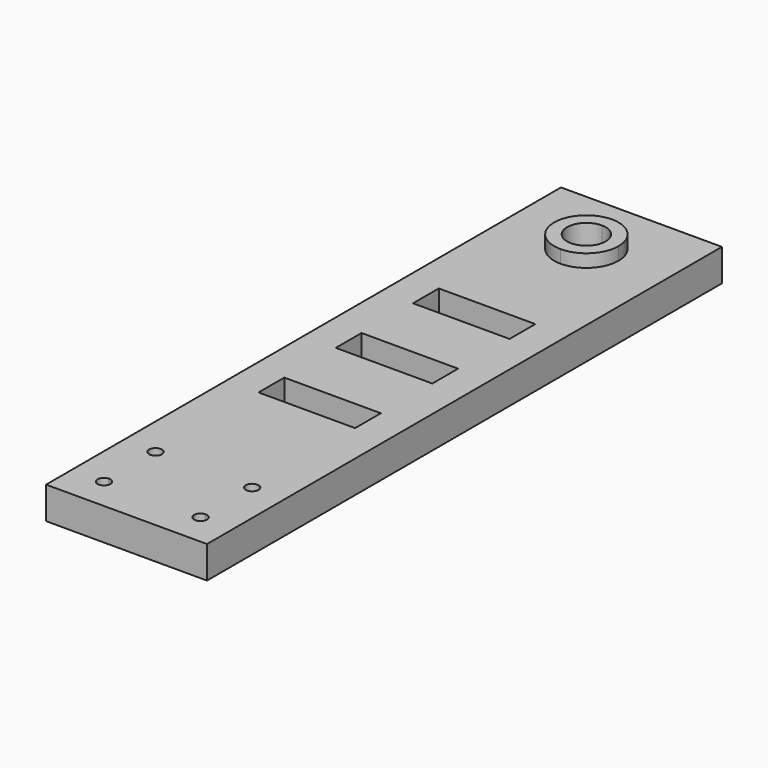
from build123d import *

# Parameters (mm, degrees)
F1_DEPTH = 5
F2_DEPTH = 7
F3_DEPTH = 1


with BuildPart() as f1:
    # F0 (on Top) → F1 (new body)
    with BuildSketch(Plane.XY):
        with BuildLine():
            Line((-12.5, -50), (0, -50))
            Line((0, -50), (0, -45))
            Line((0, -45), (-6.5, -45))
            ThreePointArc((-6.5, -45), (-8.2071067812, -45.7071067812), (-7.5, -44))
            Line((-7.5, -44), (-7.5, -35.9886))
            ThreePointArc((-7.5, -35.9886), (-8.2071067812, -34.2814932188), (-6.5, -34.9886))
            Line((-6.5, -34.9886), (0, -34.9886))
            Line((0, -34.9886), (0, -14.9886))
            Line((0, -14.9886), (-7.5, -14.9886))
            Line((-7.5, -14.9886), (-7.5, -9.9886))
            Line((-7.5, -9.9886), (0, -9.9886))
            Line((0, -9.9886), (0, 0.0114))
            Line((0, 0.0114), (-7.5, 0.0114))
            Line((-7.5, 0.0114), (-7.5, 5.0114))
            Line((-7.5, 5.0114), (0, 5.0114))
            Line((0, 5.0114), (0, 15.0114))
            Line((0, 15.0114), (-7.5, 15.0114))
            Line((-7.5, 15.0114), (-7.5, 20.0114))
            Line((-7.5, 20.0114), (0, 20.0114))
            Line((0, 20.0114), (0, 34.3023235092))
            ThreePointArc((0, 34.3023235092), (-5, 39.3023235092), (0, 44.3023235092))
            Line((0, 44.3023235092), (0, 50))
            Line((0, 50), (-12.5, 50))
            Line((-12.5, 50), (-12.5, -50))
        make_face()
        with BuildLine():
            Line((0, -50), (12.5, -50))
            Line((12.5, -50), (12.5, 50))
            Line((12.5, 50), (0, 50))
            Line((0, 50), (0, 44.3023235092))
            ThreePointArc((0, 44.3023235092), (3.5355339059, 42.8378574152), (5, 39.3023235092))
            ThreePointArc((5, 39.3023235092), (3.5355339059, 35.7667896033), (0, 34.3023235092))
            Line((0, 34.3023235092), (0, 20.0114))
            Line((0, 20.0114), (7.5, 20.0114))
            Line((7.5, 20.0114), (7.5, 15.0114))
            Line((7.5, 15.0114), (0, 15.0114))
            Line((0, 15.0114), (0, 5.0114))
            Line((0, 5.0114), (7.5, 5.0114))
            Line((7.5, 5.0114), (7.5, 0.0114))
            Line((7.5, 0.0114), (0, 0.0114))
            Line((0, 0.0114), (0, -9.9886))
            Line((0, -9.9886), (7.5, -9.9886))
            Line((7.5, -9.9886), (7.5, -14.9886))
            Line((7.5, -14.9886), (0, -14.9886))
            Line((0, -14.9886), (0, -34.9886))
            Line((0, -34.9886), (6.5, -34.9886))
            ThreePointArc((6.5, -34.9886), (7.5, -33.9886), (8.5, -34.9886))
            ThreePointArc((8.5, -34.9886), (8.2071067812, -35.6957067812), (7.5, -35.9886))
            Line((7.5, -35.9886), (7.5, -44))
            ThreePointArc((7.5, -44), (8.2071067812, -44.2928932188), (8.5, -45))
            ThreePointArc((8.5, -45), (7.5, -46), (6.5, -45))
            Line((6.5, -45), (0, -45))
            Line((0, -45), (0, -50))
        make_face()
        with BuildLine():
            Line((0, -34.9886), (0, -45))
            Line((0, -45), (6.5, -45))
            ThreePointArc((6.5, -45), (6.7928932188, -44.2928932188), (7.5, -44))
            Line((7.5, -44), (7.5, -35.9886))
            ThreePointArc((7.5, -35.9886), (6.7928932188, -35.6957067812), (6.5, -34.9886))
            Line((6.5, -34.9886), (0, -34.9886))
        make_face()
        with BuildLine():
            Line((-6.5, -45), (0, -45))
            Line((0, -45), (0, -34.9886))
            Line((0, -34.9886), (-6.5, -34.9886))
            ThreePointArc((-6.5, -34.9886), (-6.7928932188, -35.6957067812), (-7.5, -35.9886))
            Line((-7.5, -35.9886), (-7.5, -44))
            ThreePointArc((-7.5, -44), (-6.7928932188, -44.2928932188), (-6.5, -45))
        make_face()
    extrude(amount=F1_DEPTH)

    # F0 (on Top) → F2 (join)
    with BuildSketch(Plane.XY):
        with BuildLine():
            Line((0, 42.3023235092), (0, 44.3023235092))
            ThreePointArc((0, 44.3023235092), (-5, 39.3023235092), (0, 34.3023235092))
            Line((0, 34.3023235092), (0, 36.3023235092))
            ThreePointArc((0, 36.3023235092), (-3, 39.3023235092), (0, 42.3023235092))
        make_face()
        with BuildLine():
            ThreePointArc((5, 39.3023235092), (3.5355339059, 42.8378574152), (0, 44.3023235092))
            Line((0, 44.3023235092), (0, 42.3023235092))
            ThreePointArc((0, 42.3023235092), (2.1213203436, 41.4236438528), (3, 39.3023235092))
            ThreePointArc((3, 39.3023235092), (2.1213203436, 37.1810031657), (0, 36.3023235092))
            Line((0, 36.3023235092), (0, 34.3023235092))
            ThreePointArc((0, 34.3023235092), (3.5355339059, 35.7667896033), (5, 39.3023235092))
        make_face()
    extrude(amount=F2_DEPTH)

    # F0 (on Top) → F3 (join)
    with BuildSketch(Plane.XY):
        with BuildLine():
            Line((0, 41.8023235092), (0, 42.3023235092))
            ThreePointArc((0, 42.3023235092), (-3, 39.3023235092), (0, 36.3023235092))
            Line((0, 36.3023235092), (0, 36.8023235092))
            ThreePointArc((0, 36.8023235092), (-2.5, 39.3023235092), (0, 41.8023235092))
        make_face()
        with BuildLine():
            ThreePointArc((3, 39.3023235092), (2.1213203436, 41.4236438528), (0, 42.3023235092))
            Line((0, 42.3023235092), (0, 41.8023235092))
            ThreePointArc((0, 41.8023235092), (1.767766953, 41.0700904622), (2.5, 39.3023235092))
            ThreePointArc((2.5, 39.3023235092), (1.767766953, 37.5345565563), (0, 36.8023235092))
            Line((0, 36.8023235092), (0, 36.3023235092))
            ThreePointArc((0, 36.3023235092), (2.1213203436, 37.1810031657), (3, 39.3023235092))
        make_face()
    extrude(amount=F3_DEPTH)


solid = f1.part
